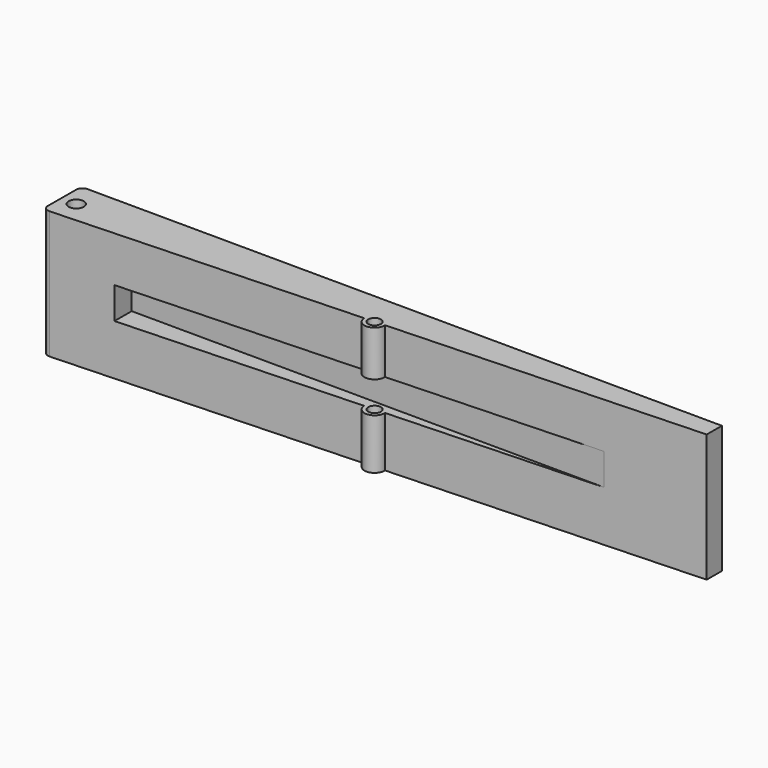
from build123d import *

# Parameters (mm, degrees)
F0_R     = 6
F1_DEPTH = 101
F2_R     = 5
F4_START = -55
F3_W     = 4.994883243
F3_H     = 25
F3_W_2   = 5.9151866052
F3_W_3   = 8.303230216
F4_DEPTH = 453


# Not quite as in the source:
# - a feature names something its author has since deleted; it is built from what else it names


with BuildPart() as f1:
    # F0 (on Top) → F1 (new body)
    with BuildSketch(Plane.XY):
        with BuildLine():
            Line((254.0328107559, 6.2914491919), (-253.9614388373, 8.7085508081))
            Line((-253.9614388373, 8.7085508081), (-254.1422456511, -29.2910190433))
            Line((-254.1422456511, -29.2910190433), (-8.0838477514, -19.3235865814))
            ThreePointArc((-8.0838477514, -19.3235865814), (-0.4142050626, -11.0063405813), (7.9030409375, -18.67598327))
            Line((7.9030409375, -18.67598327), (253.9614388373, -8.7085508081))
            Line((253.9614388373, -8.7085508081), (254.0328107559, 6.2914491919))
        make_face()
        with Locations((-241.9818616233, -11.1859360032)):
            Circle(F0_R, mode=Mode.SUBTRACT)
        with BuildLine():
            ThreePointArc((7.9030409375, -18.67598327), (-0.4142050626, -11.0063405813), (-8.0838477514, -19.3235865814))
            Line((-8.0838477514, -19.3235865814), (-5.0863061222, -19.2021609605))
            ThreePointArc((-5.0863061222, -19.2021609605), (-0.2927794417, -14.0038822105), (4.9054993084, -18.7974088909))
            Line((4.9054993084, -18.7974088909), (7.9030409375, -18.67598327))
        make_face()
        with BuildLine():
            Line((-5.0863061222, -19.2021609605), (-8.0838477514, -19.3235865814))
            ThreePointArc((-8.0838477514, -19.3235865814), (0.0715305988, -26.9981458439), (7.9095965931, -18.9997849257))
            ThreePointArc((7.9095965931, -18.9997849257), (7.9079575113, -18.83785092), (7.9030409375, -18.67598327))
            Line((7.9030409375, -18.67598327), (4.9054993084, -18.7974088909))
            ThreePointArc((4.9054993084, -18.7974088909), (4.908572167, -18.8985761721), (4.9095965931, -18.9997849257))
            ThreePointArc((4.9095965931, -18.9997849257), (0.0108053467, -23.9987604996), (-5.0863061222, -19.2021609605))
        make_face()
    extrude(amount=F1_DEPTH)

    # F2
    f2_edges = [f1.edges().sort_by_distance(p)[0] for p in [
        (-254.142246, -29.291019, 50.5),
        (-253.961439, 8.708551, 50.5),
    ]]
    fillet(f2_edges, radius=F2_R)

    # F3 (on face) → F4 (cut)
    with BuildSketch(Plane(origin=(-253.9971247966, 1.2085508081, 0), x_dir=(-0.004758074, -0.9999886803, 0), z_dir=(-0.9999886803, 0.004758074, 0)).offset(F4_START)):
        with Locations((27.7658584427, 52.5)):
            Rectangle(F3_W, F3_H)
        with Locations((22.3108235186, 52.5)):
            Rectangle(F3_W_2, F3_H)
        with Locations((15.201615108, 52.5)):
            Rectangle(F3_W_3, F3_H)
    extrude(amount=-F4_DEPTH, mode=Mode.SUBTRACT)


solid = f1.part
